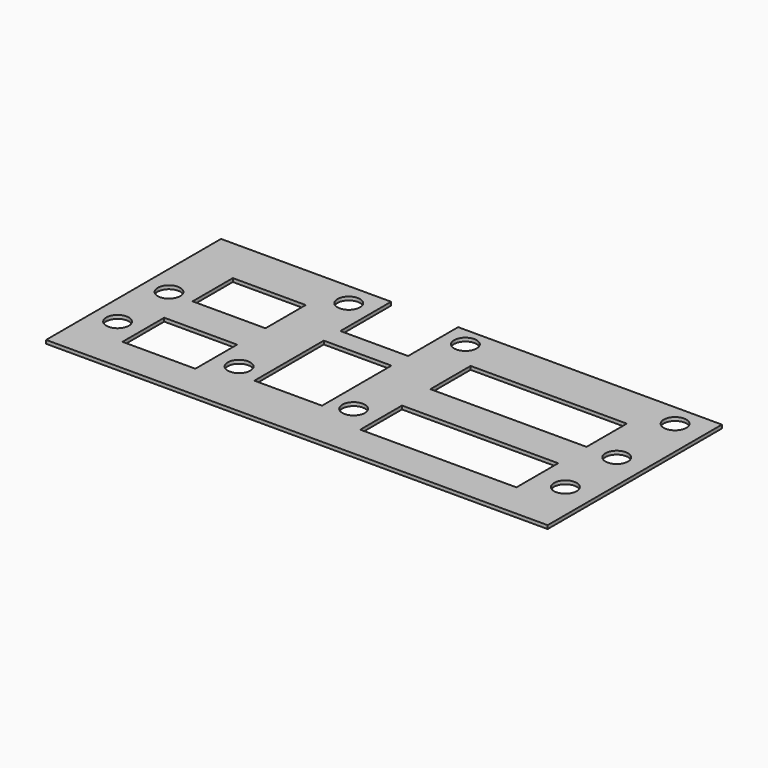
from build123d import *

# Parameters (mm, degrees)
F0_R     = 3.25
F0_W     = 21
F0_H     = 10.2114447155
F0_W_2   = 19.5
F0_H_2   = 5.9798656802
F0_W_3   = 45
F1_DEPTH = 1


# Not quite as in the source:
# - a feature names something its author has since deleted; it is built from what else it names


with BuildPart() as f1:
    # F0 (on Top) → F1 (new body)
    with BuildSketch(Plane.XY):
        Polygon((85.2658590674, -26.4641552444), (85.2658590674, 13.2858447556), (68.2658590674, 13.2858447556), (68.2658590674, -1.2141552444), (68.2658590674, -11.42559996), (68.2658590674, -26.4641552444), (23.2658590674, -26.4641552444), (9.2658590674, -26.4641552444), (9.2658590674, -22.7141552444), (-10.2341409326, -22.7141552444), (-10.2341409326, -26.4641552444), (-24.2341409326, -26.4641552444), (-45.2341409326, -26.4641552444), (-45.2341409326, -11.42559996), (-45.2341409326, -1.2141552444), (-45.2341409326, 13.2858447556), (-59.2341409326, 13.2858447556), (-59.2341409326, -26.4641552444), (-59.2341409326, -36.4641552444), (-24.2341409326, -36.4641552444), (85.2658590674, -36.4641552444), align=None)
        with Locations((-52.2341409326, -19.4641552444)):
            Circle(F0_R, mode=Mode.SUBTRACT)
        with Locations((76.7658590674, -19.4641552444)):
            Circle(F0_R, mode=Mode.SUBTRACT)
        with Locations((-52.2341409326, -0.9641552444)):
            Circle(F0_R, mode=Mode.SUBTRACT)
        with Locations((76.7658590674, -0.9641552444)):
            Circle(F0_R, mode=Mode.SUBTRACT)
        with Locations((-34.7341409326, -6.3198776022)):
            Rectangle(F0_W, F0_H)
        with Locations((-0.4841409326, 5.2757775957)):
            Rectangle(F0_W_2, F0_H_2)
        with Locations((45.7658590674, -6.3198776022)):
            Rectangle(F0_W_3, F0_H)
        Polygon((-24.2341409326, 13.2858447556), (-10.2341409326, 13.2858447556), (-10.2341409326, 26.5358447556), (-59.2341409326, 26.5358447556), (-59.2341409326, 13.2858447556), (-45.2341409326, 13.2858447556), align=None)
        with Locations((-17.2341409326, 20.0358447556)):
            Circle(F0_R, mode=Mode.SUBTRACT)
        Polygon((85.2658590674, 13.2858447556), (85.2658590674, 26.2858447556), (9.2658590674, 26.2858447556), (9.2658590674, 13.2858447556), (23.2658590674, 13.2858447556), (68.2658590674, 13.2858447556), align=None)
        with Locations((15.7658590674, 20.7858447556)):
            Circle(F0_R, mode=Mode.SUBTRACT)
        with Locations((76.7658590674, 20.0358447556)):
            Circle(F0_R, mode=Mode.SUBTRACT)
        Polygon((-10.2341409326, 2.2858447556), (-10.2341409326, 8.2657104358), (-10.2341409326, 13.2858447556), (-24.2341409326, 13.2858447556), (-24.2341409326, -1.2141552444), (-24.2341409326, -11.42559996), (-24.2341409326, -26.4641552444), (-10.2341409326, -26.4641552444), (-10.2341409326, -22.7141552444), align=None)
        with Locations((-17.2341409326, -19.4641552444)):
            Circle(F0_R, mode=Mode.SUBTRACT)
        Polygon((23.2658590674, 13.2858447556), (9.2658590674, 13.2858447556), (9.2658590674, 8.2657104358), (9.2658590674, 2.2858447556), (9.2658590674, -22.7141552444), (9.2658590674, -26.4641552444), (23.2658590674, -26.4641552444), (23.2658590674, -11.42559996), (23.2658590674, -1.2141552444), align=None)
        with Locations((15.7658590674, -19.4641552444)):
            Circle(F0_R, mode=Mode.SUBTRACT)
    extrude(amount=F1_DEPTH)


solid = f1.part
